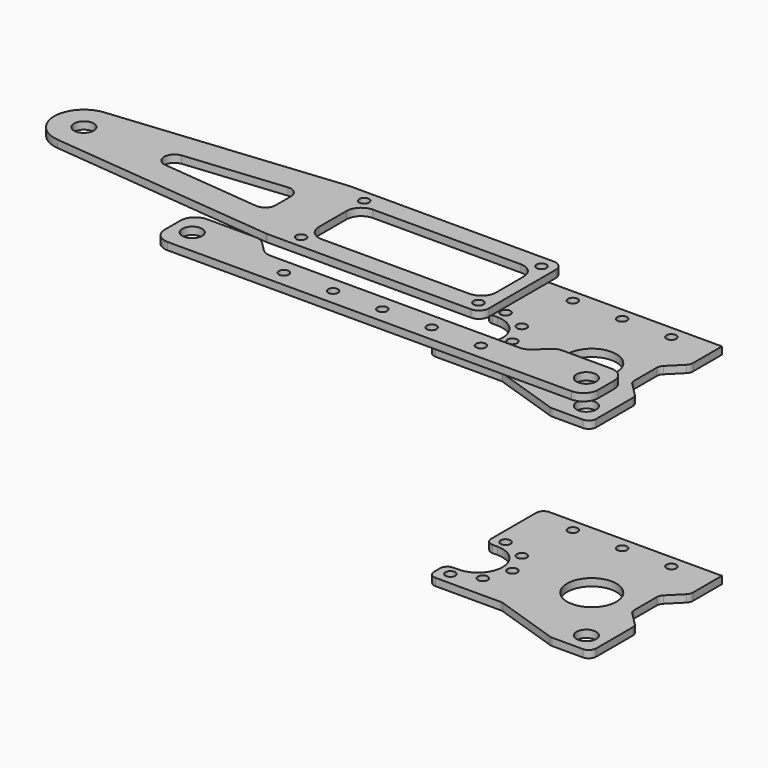
from build123d import *

# Parameters (mm, degrees)
F0_R          = 1
F0_R_2        = 2
F1_DEPTH      = 1.5
F2_W          = 36.5
F2_H          = 1.4
F3_DEPTH      = 19.75
F3_DEPTH_BACK = 1.5
F6_W          = 10
F6_H          = 39.5
F7_DEPTH      = 1.4
F10_R         = 2
F10_W         = 30
F10_H         = 2
F11_DEPTH     = 1.5
F13_W         = 95
F13_H         = 21
F13_R         = 1
F13_R_2       = 2
F14_DEPTH     = 1.5
F16_DEPTH     = 1.5
F19_R         = 5
F20_DEPTH     = 103.001
F22_DEPTH     = 1.5
F23_R         = 3
F25_DEPTH     = 1.5
F26_T1_DEPTH  = 1.9901493782
F26_T3_DEPTH  = 11.5
F27_R         = 1.5
F27_2_R       = 1.5
F29_W         = 36.5
F29_H         = 39.5
F30_DEPTH     = 3.6
F31_DEPTH     = 5
F32_R         = 1
F33_DEPTH     = 1.5


# Not quite as in the source:
# - a fillet or chamfer that OpenCascade refuses, or shapes differently, is made with other operations: its cross-section is extruded or revolved along the edge and cut away or added


with BuildPart() as f1:
    # F0 (on Top) → F1 (new body)
    with BuildSketch(Plane.XY):
        with BuildLine():
            Line((18.25, -16), (18.25, 16))
            Line((18.25, 16), (-18.25, 16))
            Line((-18.25, 16), (-18.25, 3))
            Line((-18.25, 3), (-15.75, 3))
            ThreePointArc((-15.75, 3), (-10.75, -2), (-15.75, -7))
            Line((-15.75, -7), (-18.25, -7))
            Line((-18.25, -7), (-18.25, -16))
            Line((-18.25, -16), (18.25, -16))
        make_face()
        with Locations((-15.75, -9)):
            Circle(F0_R, mode=Mode.SUBTRACT)
        with Locations((-10.8002525317, -6.9497474683)):
            Circle(F0_R, mode=Mode.SUBTRACT)
        with Locations((-8.75, -2)):
            Circle(F0_R, mode=Mode.SUBTRACT)
        with Locations((14.25, -12)):
            Circle(F0_R_2, mode=Mode.SUBTRACT)
        with Locations((-10.8002525317, 2.9497474683)):
            Circle(F0_R, mode=Mode.SUBTRACT)
        with Locations((-15.75, 5)):
            Circle(F0_R, mode=Mode.SUBTRACT)
        with Locations((-10, 14.9)):
            Circle(F0_R, mode=Mode.SUBTRACT)
        with Locations((0, 14.9)):
            Circle(F0_R, mode=Mode.SUBTRACT)
        with Locations((10, 14.9)):
            Circle(F0_R, mode=Mode.SUBTRACT)
    extrude(amount=F1_DEPTH)

    # F2 (on face) → F3 (join, two sides)
    with BuildSketch(Plane(origin=(0, 0, 0), x_dir=(1, 0, 0), z_dir=(0, 0, -1))) as f3_sk:
        with Locations((0, -16.7)):
            Rectangle(F2_W, F2_H)
    extrude(amount=F3_DEPTH)
    extrude(f3_sk.sketch, amount=-F3_DEPTH_BACK)


with BuildPart() as f5_1:
    # F5: instance of F1
    add(f1.part.mirror(Plane(origin=(0, 16.7, -19.75), x_dir=(1, 0, 0), z_dir=(0, 0, -1))))


with BuildPart() as f7_tool:
    # F6 (on face) → F7 (new body, through all)
    with BuildSketch(Plane(origin=(0, 17.4, 0), x_dir=(-1, 0, 0), z_dir=(0, 1, 0))):
        with Locations((13.25, -19.75)):
            Rectangle(F6_W, F6_H)
    extrude(amount=-F7_DEPTH)


with BuildPart() as f1_1:
    add(f1.part)

    # F7: cut by f7_tool
    add(f7_tool.part, mode=Mode.SUBTRACT)


with BuildPart() as f5_1_1:
    add(f5_1.part)

    # F7: cut by f7_tool
    add(f7_tool.part, mode=Mode.SUBTRACT)


with BuildPart() as f11:
    # F10 (on offset) → F11 (new body)
    with BuildSketch(Plane.XY.offset(5)):
        Polygon((-40.75, -7), (-69.75, -7), (-69.75, -17), (18.25, -17), (18.25, -7), (-10.75, -7), (-10.75, -9), (-40.75, -9), align=None)
        with Locations((-65.75, -12)):
            Circle(F10_R, mode=Mode.SUBTRACT)
        with Locations((14.25, -12)):
            Circle(F10_R, mode=Mode.SUBTRACT)
        with Locations((-25.75, -8)):
            Rectangle(F10_W, F10_H)
    extrude(amount=F11_DEPTH)

    # F21 (on face) → F22 (cut, through all)
    with BuildSketch(Plane.XY.offset(6.5)):
        Polygon((4.25, -7), (-55.75, -7), (-52.25, -10.5), (-25.75, -10.5), (0.75, -10.5), align=None)
    extrude(amount=-F22_DEPTH, mode=Mode.SUBTRACT)

    # F23
    f23_edges = [f11.edges().sort_by_distance(p)[0] for p in [
        (-69.75, -7, 5.75),
        (-69.75, -17, 5.75),
        (18.25, -7, 5.75),
        (18.25, -17, 5.75),
        (-55.75, -7, 5.75),
        (-52.25, -10.5, 5.75),
        (0.75, -10.5, 5.75),
        (4.25, -7, 5.75),
    ]]
    fillet(f23_edges, radius=F23_R)

    # F32 (on face) → F33 (cut, through all)
    with BuildSketch(Plane.XY.offset(6.5)):
        with Locations((-25.75, -13.75)):
            Circle(F32_R)
        with Locations((-35.75, -13.75)):
            Circle(F32_R)
        with Locations((-45.75, -13.75)):
            Circle(F32_R)
        with Locations((-15.75, -13.75)):
            Circle(F32_R)
        with Locations((-5.75, -13.75)):
            Circle(F32_R)
    extrude(amount=-F33_DEPTH, mode=Mode.SUBTRACT)


with BuildPart() as f14:
    # F13 (on offset) → F14 (new body)
    with BuildSketch(Plane.XY.offset(10)):
        with Locations((-54.25, -2)):
            Rectangle(F13_W, F13_H)
        with Locations((-45.25, -10)):
            Circle(F13_R, mode=Mode.SUBTRACT)
        with Locations((-9.25, -10)):
            Circle(F13_R, mode=Mode.SUBTRACT)
        with Locations((-95.75, -2)):
            Circle(F13_R_2, mode=Mode.SUBTRACT)
        with Locations((-45.25, 6)):
            Circle(F13_R, mode=Mode.SUBTRACT)
        with Locations((-9.25, 6)):
            Circle(F13_R, mode=Mode.SUBTRACT)
    extrude(amount=F14_DEPTH)

    # F15 (on face) → F16 (cut, through all)
    with BuildSketch(Plane.XY.offset(11.5)):
        with BuildLine():
            ThreePointArc((-101.75, -2), (-100.1952568748, 2.0298500365), (-96.336769561, 3.9712395264))
            Line((-96.336769561, 3.9712395264), (-50.25, 8.5))
            Line((-50.25, 8.5), (-101.75, 8.5))
            Line((-101.75, 8.5), (-101.75, -2))
        make_face()
        with BuildLine():
            Line((-50.25, -12.5), (-96.336769561, -7.9712395264))
            ThreePointArc((-96.336769561, -7.9712395264), (-100.1952568748, -6.0298500365), (-101.75, -2))
            Line((-101.75, -2), (-101.75, -12.5))
            Line((-101.75, -12.5), (-50.25, -12.5))
        make_face()
        with BuildLine():
            Line((-57.5553693464, 2.0552529559), (-77.5553693464, 0.0899338343))
            ThreePointArc((-77.5553693464, 0.0899338343), (-79.45, -2), (-77.5553693464, -4.0899338343))
            Line((-77.5553693464, -4.0899338343), (-57.5553693464, -6.0552529559))
            ThreePointArc((-57.5553693464, -6.0552529559), (-55.9395524872, -5.5211590278), (-55.25, -3.9653191216))
            Line((-55.25, -3.9653191216), (-55.25, -2))
            Line((-55.25, -2), (-55.25, -0.0346808784))
            ThreePointArc((-55.25, -0.0346808784), (-55.9395524872, 1.5211590278), (-57.5553693464, 2.0552529559))
        make_face()
    extrude(amount=-F16_DEPTH, mode=Mode.SUBTRACT)

    # F24 (on face) → F25 (cut, through all)
    with BuildSketch(Plane.XY.offset(11.5)):
        with BuildLine():
            Line((-12.25, 4.5), (-42.25, 4.5))
            ThreePointArc((-42.25, 4.5), (-44.3713203436, 3.6213203436), (-45.25, 1.5))
            Line((-45.25, 1.5), (-45.25, -5.5))
            ThreePointArc((-45.25, -5.5), (-44.3713203436, -7.6213203436), (-42.25, -8.5))
            Line((-42.25, -8.5), (-12.25, -8.5))
            ThreePointArc((-12.25, -8.5), (-10.1286796564, -7.6213203436), (-9.25, -5.5))
            Line((-9.25, -5.5), (-9.25, 1.5))
            ThreePointArc((-9.25, 1.5), (-10.1286796564, 3.6213203436), (-12.25, 4.5))
        make_face()
    extrude(amount=-F25_DEPTH, mode=Mode.SUBTRACT)

    # F26: fillet of radius 2 on 4 edges, made by hand

    # F26_s2 → F26_t1 (cut)
    with BuildSketch(Plane.XY.offset(9.7549253109)):
        with BuildLine():
            ThreePointArc((-50.347559978, 8.4904131755), (-50.2498824551, 8.4976018561), (-50.1519701244, 8.5))
            Line((-50.1519701244, 8.5), (-50.25, 8.5))
            Line((-50.25, 8.5), (-50.347559978, 8.4904131755))
        make_face()
        with BuildLine():
            ThreePointArc((-50.1519701244, -12.5), (-50.2498824551, -12.4976018561), (-50.347559978, -12.4904131755))
            Line((-50.347559978, -12.4904131755), (-50.25, -12.5))
            Line((-50.25, -12.5), (-50.1519701244, -12.5))
        make_face()
    extrude(amount=F26_T1_DEPTH, mode=Mode.SUBTRACT)

    # F26_s4 → F26_t3 (cut)
    with BuildSketch(Plane.XY.offset(5)):
        with BuildLine():
            ThreePointArc((-8.75, -12.5), (-7.3357864376, -11.9142135624), (-6.75, -10.5))
            Line((-6.75, -10.5), (-6.75, -12.5))
            Line((-6.75, -12.5), (-8.75, -12.5))
        make_face()
        with BuildLine():
            ThreePointArc((-6.75, 6.5), (-7.3357864376, 7.9142135624), (-8.75, 8.5))
            Line((-8.75, 8.5), (-6.75, 8.5))
            Line((-6.75, 8.5), (-6.75, 6.5))
        make_face()
    extrude(amount=F26_T3_DEPTH, mode=Mode.SUBTRACT)


with BuildPart() as f18_1:
    # F18: instance of F1
    add(f1_1.part.mirror(Plane.XY.offset(-50)))


with BuildPart() as f20_tool:
    # F19 (on face) → F20 (new body, through all)
    with BuildSketch(Plane.XY.offset(1.5)):
        Polygon((18.25, -4.6), (18.25, 9.4), (14.75, 5.9), (14.75, 2.4), (14.75, -1.1), align=None)
        with Locations((5.75, 0)):
            Circle(F19_R)
        Polygon((-3.25, -11.5), (-18.25, -11.5), (-18.25, -16), (10.25, -16), align=None)
    extrude(amount=-F20_DEPTH)


with BuildPart() as f1_2:
    add(f1_1.part)

    # F20: cut by f20_tool
    add(f20_tool.part, mode=Mode.SUBTRACT)

    # F27
    f27_edges = [f1_2.edges().sort_by_distance(p)[0] for p in [
        (18.25, -4.6, 0.75),
        (18.25, 9.4, 0.75),
        (10.25, -16, 0.75),
        (18.25, -16, 0.75),
        (14.75, -1.1, 0.75),
        (14.75, 5.9, 0.75),
        (-18.25, 17.4, 0.75),
        (-18.25, 3, 0.75),
        (-18.25, -7, 0.75),
        (-18.25, -11.5, 0.75),
    ]]
    fillet(f27_edges, radius=F27_R)



with BuildPart() as f5_1_2:
    add(f5_1_1.part)

    # F20: cut by f20_tool
    add(f20_tool.part, mode=Mode.SUBTRACT)

    # F27#2
    f27_2_edges = [f5_1_2.edges().sort_by_distance(p)[0] for p in [
        (-18.25, -11.5, -40.25),
        (-3.25, -11.5, -40.25),
        (10.25, -16, -40.25),
        (18.25, -16, -40.25),
        (14.75, -1.1, -40.25),
        (14.75, 5.9, -40.25),
        (-18.25, 17.4, -40.25),
        (-18.25, -7, -40.25),
        (-18.25, 3, -40.25),
        (18.25, -4.6, -40.25),
        (18.25, 9.4, -40.25),
    ]]
    fillet(f27_2_edges, radius=F27_2_R)


with BuildPart() as f18_1_1:
    add(f18_1.part)

    # F20: cut by f20_tool
    add(f20_tool.part, mode=Mode.SUBTRACT)


with BuildPart() as f1_3:
    add(f1_2.part)

    add(f5_1_2.part)  # F30 merges F5_1
    # F29 (on face) → F30 (join)
    with BuildSketch(Plane.XZ.offset(-16)):
        with Locations((0, -19.75)):
            Rectangle(F29_W, F29_H)
    extrude(amount=F30_DEPTH)

    # F31 (cut): a face of the model
    f31_faces = [f1_3.faces().sort_by_distance(p)[0] for p in [
        (0, 12.4, -19.75),
    ]]
    extrude(f31_faces, amount=-F31_DEPTH, mode=Mode.SUBTRACT)


solid = Compound([f11.part, f14.part, f1_3.part])
